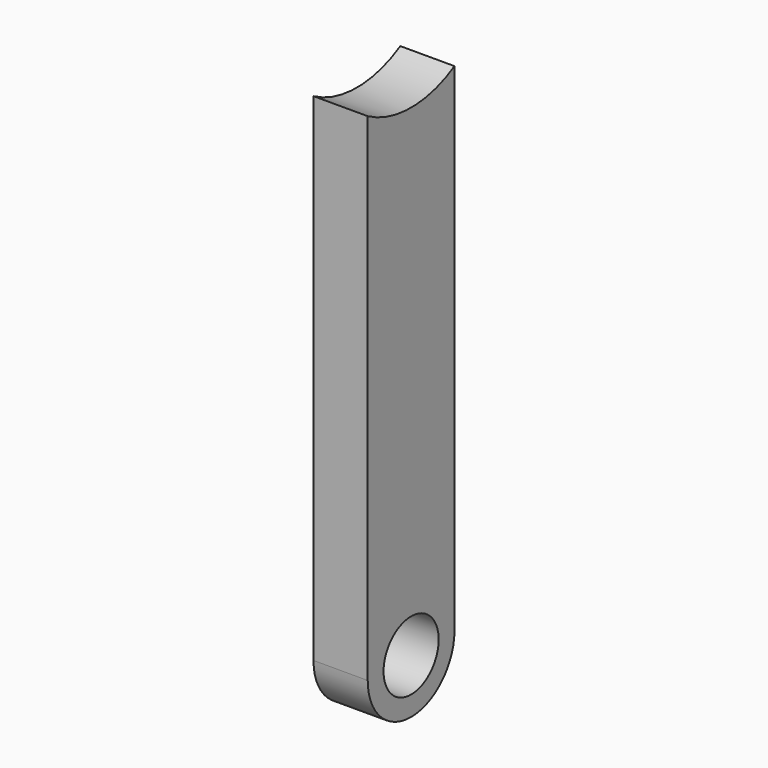
from build123d import *

# Parameters (mm, degrees)
F0_W     = 10
F0_H     = 20
F1_DEPTH = 101.6
F2_R     = 6.35
F2_R_2   = 20
F3_DEPTH = 25.4
F4_R     = 9.99999


# Not quite as in the source:
# - a fillet or chamfer is up to 0.001 mm smaller than in the source, because OpenCascade refuses the exact size


with BuildPart() as f1:
    # F0 (on Top) → F1 (new body)
    with BuildSketch(Plane.XY):
        with Locations((5, -10)):
            Rectangle(F0_W, F0_H)
    extrude(amount=F1_DEPTH)

    # F2 (on face) → F3 (cut)
    with BuildSketch(Plane(origin=(0, 0, 0), x_dir=(0, -1, 0), z_dir=(-1, 0, 0))):
        with Locations((10, 10)):
            Circle(F2_R)
        with Locations((10, 118.9205080757)):
            Circle(F2_R_2)
    extrude(amount=-F3_DEPTH, mode=Mode.SUBTRACT)

    # F4 (radius 10 in the source; OpenCascade refuses exactly that, so slightly less here)
    f4_edges = [f1.edges().sort_by_distance(p)[0] for p in [
        (5, -20, 0),
        (5, 0, 0),
    ]]
    fillet(f4_edges, radius=F4_R)


solid = f1.part
